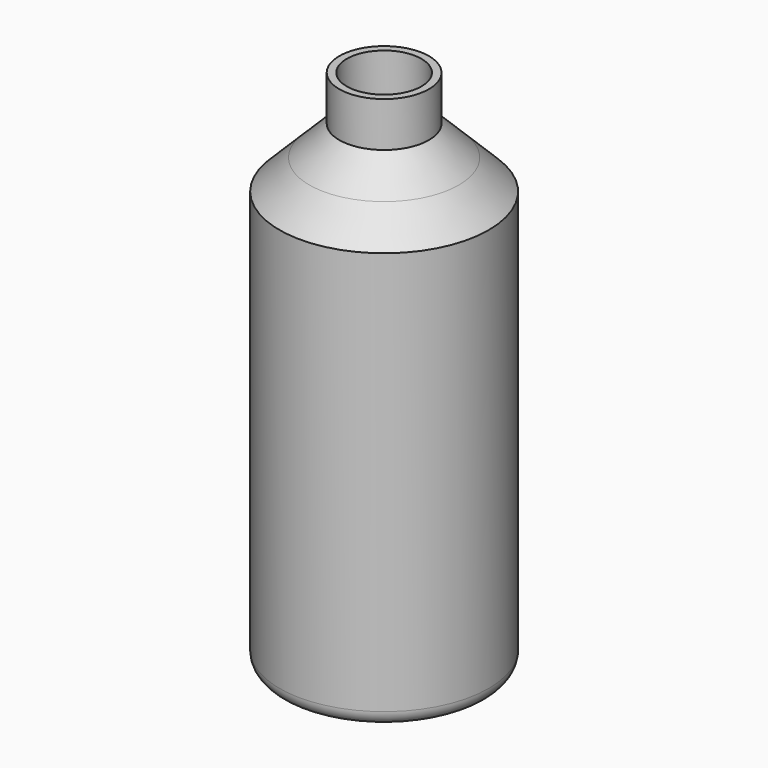
from build123d import *

# Parameters (mm, degrees)
F0_R     = 35
F1_DEPTH = 150
F2_R     = 15
F3_DEPTH = 25
F4_R     = 5
F5_R     = 15
F6_DEPTH = 20
F7_SIZE  = 9.99999
F8_T     = -2.5


# Not quite as in the source:
# - a fillet or chamfer is up to 0.001 mm smaller than in the source, because OpenCascade refuses the exact size


with BuildPart() as f1:
    # F0 (on Top) → F1 (new body)
    with BuildSketch(Plane.XY):
        Circle(F0_R)
    extrude(amount=F1_DEPTH)

    # F2 (on face) → F3 (join)
    with BuildSketch(Plane.XY.offset(150)):
        Circle(F2_R)
    extrude(amount=F3_DEPTH)

    # F4
    f4_edges = [f1.edges().sort_by_distance(p)[0] for p in [
        (-35, 0, 0),
    ]]
    fillet(f4_edges, radius=F4_R)

    # F5 (on face) → F6 (cut)
    with BuildSketch(Plane(origin=(0, 0, 0), x_dir=(1, 0, 0), z_dir=(0, 0, -1))):
        Circle(F5_R)
    extrude(amount=-F6_DEPTH, mode=Mode.SUBTRACT)

    # F7 (size 10 in the source; OpenCascade refuses exactly that, so slightly less here)
    f7_edges = [f1.edges().sort_by_distance(p)[0] for p in [
        (-35, 0, 150),
        (-15, 0, 150),
    ]]
    chamfer(f7_edges, length=F7_SIZE)

    # F8
    f8_openings = [f1.faces().sort_by_distance(p)[0] for p in [
        (0, 0, 175),
    ]]
    offset(amount=F8_T, openings=f8_openings, kind=Kind.INTERSECTION)


solid = f1.part
